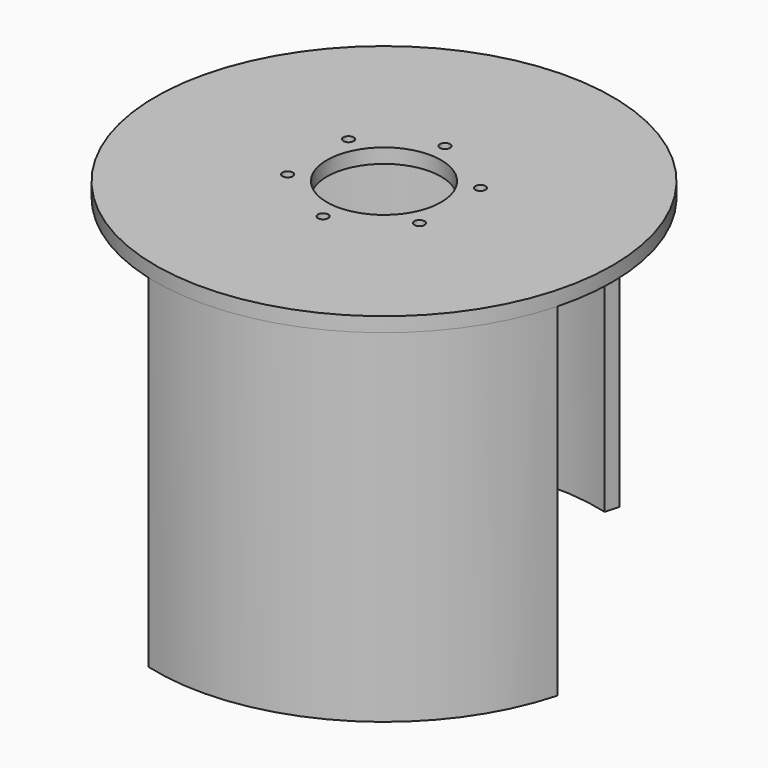
from build123d import *

# Parameters (mm, degrees)
F0_R     = 150
F0_R_2   = 3.4
F0_R_3   = 37.5
F1_DEPTH = 9.525
F3_DEPTH = 225


# Not quite as in the source:
# - a length typed as a fraction of an inch, garbled in the dataset ("3 / 203.2 mm" for 3/8 in), is restored


with BuildPart() as f1:
    # F0 (on Top) → F1 (new body)
    with BuildSketch(Plane.XY):
        Circle(F0_R)
        with Locations((-43.3012701892, -25)):
            Circle(F0_R_2, mode=Mode.SUBTRACT)
        with Locations((0, -50)):
            Circle(F0_R_2, mode=Mode.SUBTRACT)
        with Locations((43.3012701892, -25)):
            Circle(F0_R_2, mode=Mode.SUBTRACT)
        with Locations((-43.3012701892, 25)):
            Circle(F0_R_2, mode=Mode.SUBTRACT)
        Circle(F0_R_3, mode=Mode.SUBTRACT)
        with Locations((43.3012701892, 25)):
            Circle(F0_R_2, mode=Mode.SUBTRACT)
        with Locations((0, 50)):
            Circle(F0_R_2, mode=Mode.SUBTRACT)
    extrude(amount=F1_DEPTH)

    # F2 (on face) → F3 (join)
    with BuildSketch(Plane(origin=(0, 0, 0), x_dir=(1, 0, 0), z_dir=(0, 0, -1))):
        with BuildLine():
            Line((-135.688430448, -36.3576053608), (-144.8888739434, -38.8228567654))
            ThreePointArc((-144.8888739434, -38.8228567654), (-75, -129.9038105677), (38.8228567654, -144.8888739434))
            Line((38.8228567654, -144.8888739434), (36.3576053608, -135.688430448))
            ThreePointArc((36.3576053608, -135.688430448), (-70.2375, -121.6549185966), (-135.688430448, -36.3576053608))
        make_face()
        with BuildLine():
            ThreePointArc((-36.3576053608, 135.688430448), (70.2375, 121.6549185966), (135.688430448, 36.3576053608))
            Line((135.688430448, 36.3576053608), (144.8888739434, 38.8228567654))
            ThreePointArc((144.8888739434, 38.8228567654), (75, 129.9038105677), (-38.8228567654, 144.8888739434))
            Line((-38.8228567654, 144.8888739434), (-36.3576053608, 135.688430448))
        make_face()
    extrude(amount=F3_DEPTH)


solid = f1.part
